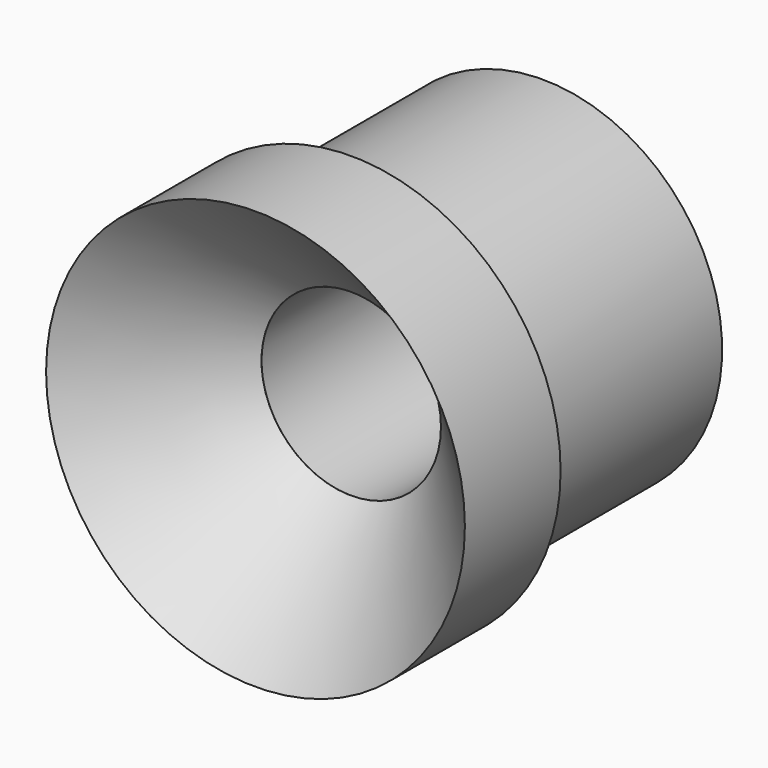
from build123d import *

# Parameters (mm, degrees)
F0_R     = 3.5
F0_R_2   = 1.5
F1_DEPTH = 2
F2_SIZE  = 1.99999
F3_R     = 3
F3_R_2   = 1.5
F4_DEPTH = 4


# Not quite as in the source:
# - a fillet or chamfer is up to 0.001 mm smaller than in the source, because OpenCascade refuses the exact size


with BuildPart() as f1:
    # F0 (on Front) → F1 (new body)
    with BuildSketch(Plane.XZ):
        Circle(F0_R)
        Circle(F0_R_2, mode=Mode.SUBTRACT)
    extrude(amount=F1_DEPTH)

    # F2 (size 2 in the source; OpenCascade refuses exactly that, so slightly less here)
    f2_edges = [f1.edges().sort_by_distance(p)[0] for p in [
        (-1.5, -2, 0),
    ]]
    chamfer(f2_edges, length=F2_SIZE)

    # F3 (on face) → F4 (join)
    with BuildSketch(Plane(origin=(0, 0, 0), x_dir=(-1, 0, 0), z_dir=(0, 1, 0))):
        Circle(F3_R)
        Circle(F3_R_2, mode=Mode.SUBTRACT)
    extrude(amount=F4_DEPTH)


solid = f1.part
